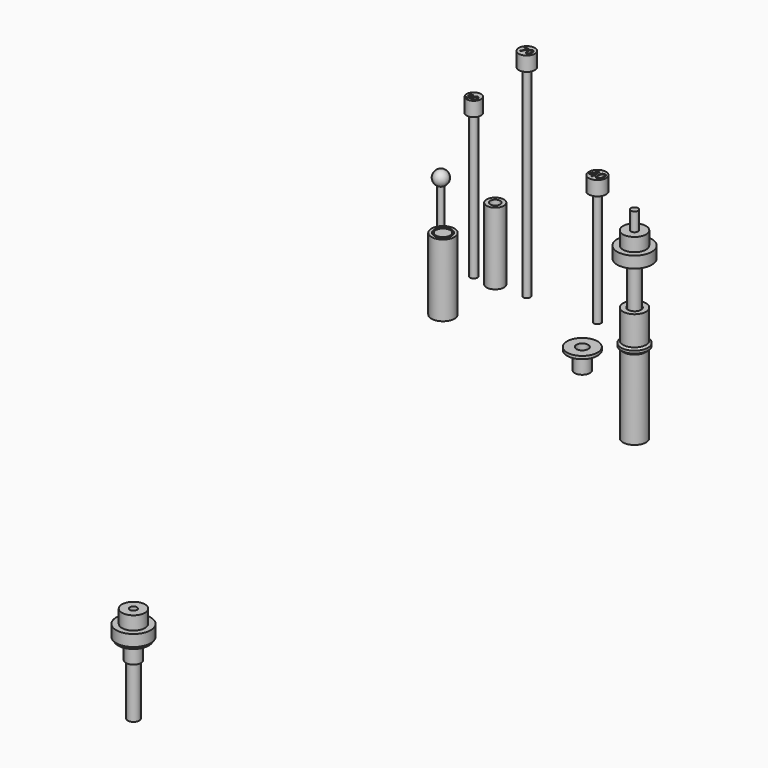
from build123d import *

# Parameters (mm, degrees)
F0_R          = 3
F0_R_2        = 1.75
F1_DEPTH      = 25
F2_R          = 1
F3_DEPTH      = 25
F6_R          = 1.25
F7_DEPTH      = 70
F15_R         = 2.7994545142
F15_R_2       = 1.25
F16_DEPTH     = 5
F17_TEXT_SIZE = 3.4524612272
F18_DEPTH     = 3
F19_R         = 1.25
F20_DEPTH     = 50
F21_R         = 2.5
F21_R_2       = 1.25
F22_DEPTH     = 5
F23_TEXT_SIZE = 3.1935266352
F24_DEPTH     = 2.5
F25_R         = 1.25
F26_DEPTH     = 40
F27_R         = 3.0170793683
F27_R_2       = 1.25
F28_DEPTH     = 5
F29_TEXT_SIZE = 4.4252524579
F30_DEPTH     = 2.5
F31_R         = 2.5
F32_DEPTH     = 25
F31_R_2       = 4
F31_R_3       = 3
F33_R         = 4
F33_R_2       = 2.25
F34_DEPTH     = 10
F35_DEPTH     = 30
F36_R         = 1.25
F37_DEPTH     = 70
F38_R         = 4.6521571756
F38_R_2       = 1.7232428156
F39_DEPTH     = 2.5
F40_S5_R      = 4
F40_T6_DEPTH  = 8
F40_S11_R     = 4
F40_T12_DEPTH = 8


# Not quite as in the source:
# - a fillet or chamfer that OpenCascade refuses, or shapes differently, is made with other operations: its cross-section is extruded or revolved along the edge and cut away or added
# - Text() gives the source's letters only with a copy of the font that has no kerning and outlines rounded to 1/6400 em; it was checked with that copy


with BuildPart() as f1:
    # F0 (on Top) → F1 (new body)
    with BuildSketch(Plane.XY):
        Circle(F0_R)
        Circle(F0_R_2, mode=Mode.SUBTRACT)
    extrude(amount=F1_DEPTH)


with BuildPart() as f3:
    # F2 (on Top) → F3 (new body)
    with BuildSketch(Plane.XY):
        with Locations((-18.9045504432, 0)):
            Circle(F2_R)
    extrude(amount=F3_DEPTH)

    # F4 (on Front) → F5 (revolve)
    with BuildSketch(Plane.XZ):
        with BuildLine():
            Line((-18.9066084971, 24.0000001342), (-18.9066084971, 28.9999998658))
            ThreePointArc((-18.9066084971, 28.9999998658), (-21.4074277878, 26.5), (-18.9066084971, 24.0000001342))
        make_face()
    revolve(axis=Axis((-18.9066084971, 0, 25.0019133628), (0, 0, 1)))


with BuildPart() as f7:
    # F6 (on Top) → F7 (new body)
    with BuildSketch(Plane.XY):
        with Locations((10.984466734, 0)):
            Circle(F6_R)
    extrude(amount=F7_DEPTH)

    # F15 (on face) → F16 (join)
    with BuildSketch(Plane.XY.offset(70)):
        with Locations((10.984466734, 0)):
            Circle(F15_R)
        with Locations((10.984466734, 0)):
            Circle(F15_R_2, mode=Mode.SUBTRACT)
        with Locations((10.984466734, 0)):
            Circle(F15_R_2)
    extrude(amount=F16_DEPTH)

    # F17 (on face) → F18 (cut)
    with BuildSketch(Plane.XY.offset(75)):
        with Locations((8.9993090182, -1.2064912674)):
            Text('70', F17_TEXT_SIZE, font='Open Sans', text_align=(TextAlign.LEFT, TextAlign.BOTTOM))
    extrude(amount=-F18_DEPTH, mode=Mode.SUBTRACT)


with BuildPart() as f10:
    # F9 (on offset) → F10 (revolve)
    with BuildSketch(Plane.YZ.offset(50)):
        Polygon((-4, 25), (-4, 0), (-3.25, 0), (-3.25, 33.6408875883), (-6, 33.6408875883), (-6, 28.9735510945), (-8, 28.9735510945), (-8, 25), align=None)
    revolve(axis=Axis((50, -2, 22.5835368037), (0, 0, 1)))


with BuildPart() as f12:
    # F11 (on offset) → F12 (revolve)
    with BuildSketch(Plane.YZ.offset(50)):
        Polygon((-27.3364575086, 6.15), (-27.3364575086, 0), (-26.7364575086, 0), (-26.7364575086, 7.15), (-29.9864575086, 7.15), (-29.9864575086, 6.15), align=None)
    revolve(axis=Axis((50, -24.6864575086, 0.9171422474), (0, 0, -1)))


with BuildPart() as f14:
    # F13 (on offset) → F14 (revolve)
    with BuildSketch(Plane.YZ.offset(50)):
        Polygon((-221.6443974972, -9.4253822612), (-221.6443974972, -27.2753822612), (-220.8943974972, -27.2753822612), (-220.8943974972, 6.3655053271), (-223.6443974972, 6.3655053271), (-223.6443974972, 1.6981688334), (-225.6443974972, 1.6981688334), (-225.6443974972, -2.2753822612), (-224.9443974972, -2.2753822612), (-224.9443974972, -3.2753822612), (-222.2943974972, -3.2753822612), (-222.2943974972, -9.4253822612), align=None)
    revolve(axis=Axis((50, -219.6443974972, 25.8106369905), (0, 0, 1)))


with BuildPart() as f20:
    # F19 (on Top) → F20 (new body)
    with BuildSketch(Plane.XY):
        with Locations((-7.4660787519, 0)):
            Circle(F19_R)
    extrude(amount=F20_DEPTH)

    # F21 (on face) → F22 (join)
    with BuildSketch(Plane.XY.offset(50)):
        with Locations((-7.4660787519, 0)):
            Circle(F21_R)
        with Locations((-7.4660787519, 0)):
            Circle(F21_R_2, mode=Mode.SUBTRACT)
        with Locations((-7.4660787519, 0)):
            Circle(F21_R_2)
    extrude(amount=F22_DEPTH)

    # F23 (on face) → F24 (cut)
    with BuildSketch(Plane.XY.offset(55)):
        with Locations((-9.3191681332, -1.6849098393)):
            Text('50', F23_TEXT_SIZE, font='Open Sans', text_align=(TextAlign.LEFT, TextAlign.BOTTOM))
    extrude(amount=-F24_DEPTH, mode=Mode.SUBTRACT)


with BuildPart() as f26:
    # F25 (on Top) → F26 (new body)
    with BuildSketch(Plane.XY):
        with Locations((35.4971538786, 0)):
            Circle(F25_R)
    extrude(amount=F26_DEPTH)

    # F27 (on face) → F28 (join)
    with BuildSketch(Plane.XY.offset(40)):
        with Locations((35.4971538786, 0)):
            Circle(F27_R)
        with Locations((35.4971538786, 0)):
            Circle(F27_R_2, mode=Mode.SUBTRACT)
        with Locations((35.4971538786, 0)):
            Circle(F27_R_2)
    extrude(amount=F28_DEPTH)

    # F29 (on face) → F30 (cut)
    with BuildSketch(Plane.XY.offset(45)):
        with Locations((32.9469665885, -1.5640655765)):
            Text('40', F29_TEXT_SIZE, font='Open Sans', text_align=(TextAlign.LEFT, TextAlign.BOTTOM))
    extrude(amount=-F30_DEPTH, mode=Mode.SUBTRACT)


with BuildPart() as f32:
    # F31 (on Top) → F32 (new body)
    with BuildSketch(Plane.XY):
        with Locations((0, -22.710137567)):
            Circle(F31_R)
    extrude(amount=F32_DEPTH)


with BuildPart() as f32b:
    # F31 (on Top) → F32, piece 2 (new body)
    with BuildSketch(Plane.XY):
        with Locations((0, -22.710137567)):
            Circle(F31_R_2)
        with Locations((0, -22.710137567)):
            Circle(F31_R_3, mode=Mode.SUBTRACT)
    extrude(amount=F32_DEPTH)


with BuildPart() as f34:
    # F33 (on Top) → F34 (new body)
    with BuildSketch(Plane.XY):
        with Locations((50.0034019351, -2.0053146873)):
            Circle(F33_R)
        with Locations((50.0034019351, -2.0053146873)):
            Circle(F33_R_2, mode=Mode.SUBTRACT)
    extrude(amount=F34_DEPTH)

    # F33 (on Top) → F35 (join)
    with BuildSketch(Plane.XY):
        with Locations((50.0034019351, -2.0053146873)):
            Circle(F33_R)
        with Locations((50.0034019351, -2.0053146873)):
            Circle(F33_R_2, mode=Mode.SUBTRACT)
    extrude(amount=-F35_DEPTH)

    # F38 (on Top) → F39 (join)
    with BuildSketch(Plane.XY):
        with Locations((50.0034019351, -2.0053146873)):
            Circle(F38_R)
        with Locations((50.0034019351, -2.0053146873)):
            Circle(F38_R_2, mode=Mode.SUBTRACT)
    extrude(amount=-F39_DEPTH)

    # F40: chamfer of 0.8 on 2 edges, made by hand


with BuildPart() as f37:
    # F36 (on face) → F37 (new body)
    with BuildSketch(Plane(origin=(0, 0, -30), x_dir=(1, 0, 0), z_dir=(0, 0, -1))):
        with Locations((50.0034019351, 2.0053146873)):
            Circle(F36_R)
    extrude(amount=-F37_DEPTH)


with BuildPart() as f40_tool2:
    # F40_s3 → F40_t4 (revolve)
    with BuildSketch(Plane.XZ.offset(2.0053146873)):
        Polygon((54.6555591107, -1.7), (53.8555591107, -2.5), (54.6555591107, -2.5), align=None)
    revolve(axis=Axis((50.0034019351, -2.0053146873, -2.5), (0, 0, 1)))

    # F40_s5 → F40_t6 (cut, symmetric)
    with BuildSketch(Plane.XY.offset(-2.1)):
        with Locations((50.0034019351, -2.0053146873)):
            Circle(F40_S5_R)
    extrude(amount=F40_T6_DEPTH, both=True, mode=Mode.SUBTRACT)


with BuildPart() as f34_1:
    add(f34.part)

    # F40_t1: cut F40_tool2
    add(f40_tool2.part, mode=Mode.SUBTRACT)


with BuildPart() as f40_tool8:
    # F40_s9 → F40_t10 (revolve)
    with BuildSketch(Plane.XZ.offset(2.0053146873)):
        Polygon((53.8555591107, 0), (54.6555591107, -0.8), (54.6555591107, 0), align=None)
    revolve(axis=Axis((50.0034019351, -2.0053146873, 0), (0, 0, 1)))

    # F40_s11 → F40_t12 (cut, symmetric)
    with BuildSketch(Plane.XY.offset(-0.4)):
        with Locations((50.0034019351, -2.0053146873)):
            Circle(F40_S11_R)
    extrude(amount=F40_T12_DEPTH, both=True, mode=Mode.SUBTRACT)


with BuildPart() as f34_2:
    add(f34_1.part)

    # F40_t7: cut F40_tool8
    add(f40_tool8.part, mode=Mode.SUBTRACT)

    # F41: fillet of radius 1 on 1 edges, made by hand

    # F41_s1 → F41_t2 (revolve, cut)
    with BuildSketch(Plane.XZ.offset(2.0053146873)):
        with BuildLine():
            ThreePointArc((51.7266447507, -1.6190679723), (51.8683782374, -2.1322722125), (52.2534019351, -2.5))
            Line((52.2534019351, -2.5), (51.7266447507, -2.5))
            Line((51.7266447507, -2.5), (51.7266447507, -1.6190679723))
        make_face()
    revolve(axis=Axis((50.0034019351, -2.0053146873, -2.5), (0, 0, 1)), mode=Mode.SUBTRACT)


solid = Compound([f1.part, f3.part, f7.part, f10.part, f12.part, f14.part, f20.part, f26.part, f32.part, f32b.part, f37.part, f34_2.part])
